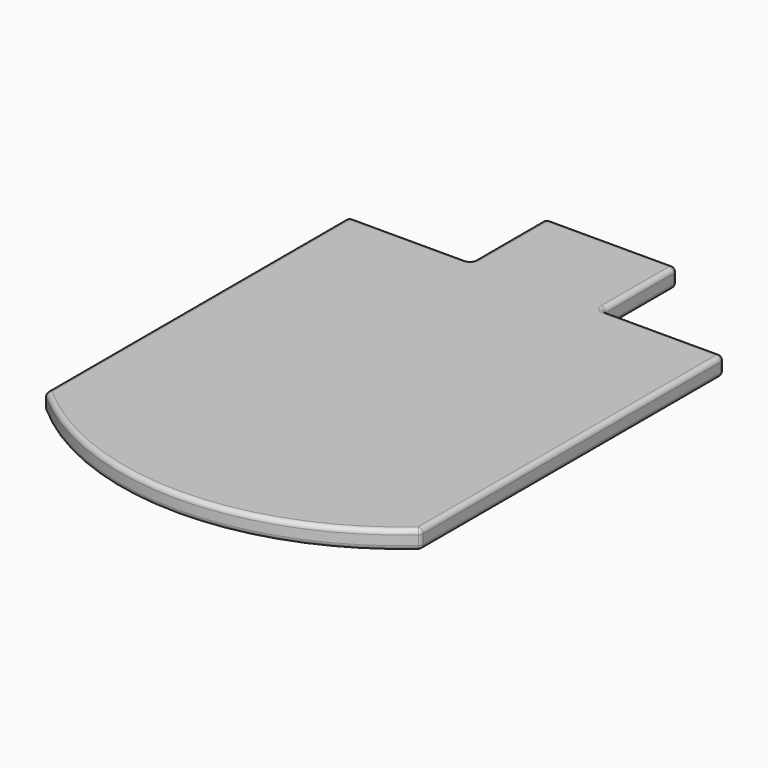
from build123d import *

# Parameters (mm, degrees)
F1_DEPTH = 20
F2_R     = 300
F3_DEPTH = 20.001
F4_R     = 5


with BuildPart() as f1:
    # F0 (on Top) → F1 (new body)
    with BuildSketch(Plane.XY):
        Polygon((70, 0), (-70, 0), (-70, -100), (-200, -100), (-200, -600), (200, -600), (200, -100), (70, -100), align=None)
    extrude(amount=F1_DEPTH)

    # F2 (on face) → F3 (intersect, through all)
    with BuildSketch(Plane.XY.offset(20)):
        with Locations((0, -280)):
            Circle(F2_R)
    extrude(amount=-F3_DEPTH, mode=Mode.INTERSECT)

    # F4
    f4_edges = [f1.edges().sort_by_distance(p)[0] for p in [
        (70, -50, 20),
        (135, -100, 20),
        (200, -301.803399, 20),
        (0, -580, 20),
        (-200, -301.803399, 20),
        (-135, -100, 20),
        (-70, -50, 20),
        (0, 0, 20),
        (70, 0, 10),
        (-70, 0, 10),
        (0, 0, 0),
        (70, -50, 0),
        (135, -100, 0),
        (200, -301.803399, 0),
        (0, -580, 0),
        (-200, -301.803399, 0),
        (-135, -100, 0),
        (-70, -50, 0),
        (200, -100, 10),
        (70, -100, 10),
        (-70, -100, 10),
        (-200, -100, 10),
        (200, -503.606798, 10),
        (-200, -503.606798, 10),
    ]]
    fillet(f4_edges, radius=F4_R)


solid = f1.part
